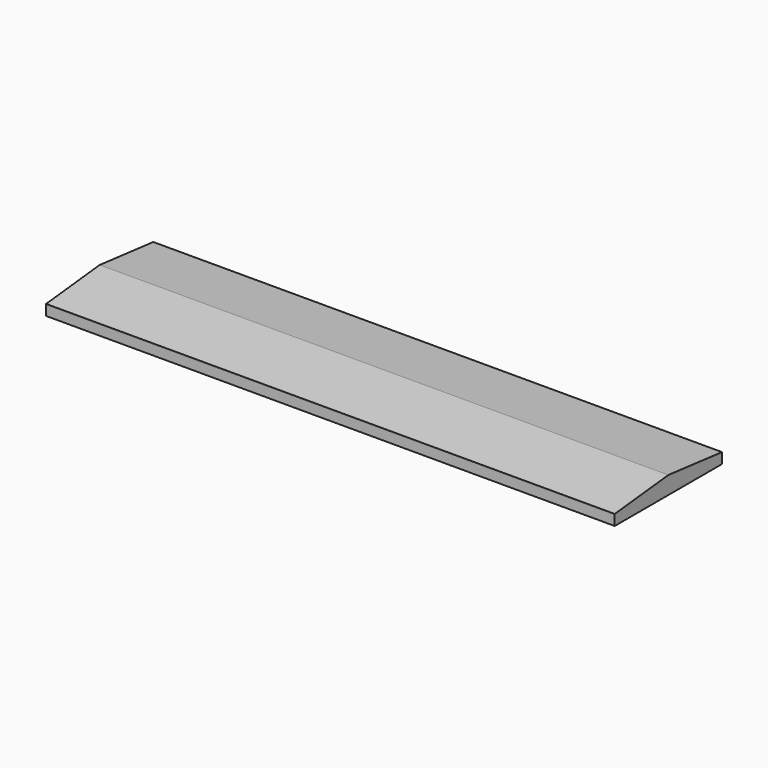
from build123d import *

# Parameters (mm, degrees)
F0_W          = 39250
F0_H          = 9250
F1_DEPTH      = 150
F2_W          = 39250
F2_H          = 9250
F2_W_2        = 38950
F2_H_2        = 8950
F3_DEPTH      = 570
F5_DEPTH      = 39250.001
F7_DEPTH      = 50
F7_DEPTH_BACK = 39300
F9_DEPTH      = 150
F11_DEPTH     = 150
F12_W         = 266.9223773158
F12_H         = 1000
F13_DEPTH     = 1220.2764139782
F14_W         = 44695.1484680176
F14_H         = 14306.3936233521
F14_W_2       = 39250
F14_H_2       = 9250
F15_DEPTH     = 1220.2764139782
F17_DEPTH     = 38950


with BuildPart() as f1:
    # F0 (on Top) → F1 (new body)
    with BuildSketch(Plane.XY):
        with Locations((19625, -4625)):
            Rectangle(F0_W, F0_H)
    extrude(amount=F1_DEPTH)

    # F2 (on face) → F3 (join)
    with BuildSketch(Plane.XY.offset(150)):
        with Locations((19625, -4625)):
            Rectangle(F2_W, F2_H)
        with Locations((19625, -4625)):
            Rectangle(F2_W_2, F2_H_2, mode=Mode.SUBTRACT)
    extrude(amount=F3_DEPTH)

    # F4 (on face) → F5 (cut, through all)
    with BuildSketch(Plane(origin=(0, 0, 0), x_dir=(0, -1, 0), z_dir=(-1, 0, 0))):
        Polygon((-659.6078069495, 614.5653377715), (4625, 1170), (1956.3378095627, 2374.1724491119), align=None)
        Polygon((7293.6621904373, 2374.1724491119), (4625, 1170), (9909.6078069495, 614.5653377715), align=None)
    extrude(amount=-F5_DEPTH, mode=Mode.SUBTRACT)

    # F8 (on face) → F9 (join)
    with BuildSketch(Plane.YZ.offset(39250)):
        Polygon((-8906.4640044002, 720), (-343.5359955999, 720), (-4625, 1170), align=None)
    extrude(amount=-F9_DEPTH)

    # F10 (on face) → F11 (join)
    with BuildSketch(Plane(origin=(0, 0, 0), x_dir=(0, -1, 0), z_dir=(-1, 0, 0))):
        Polygon((4625, 1170), (343.5359955998, 720), (8906.4640044001, 720), align=None)
    extrude(amount=-F11_DEPTH)


with BuildPart() as f7:
    # F6 (on face) → F7 (new body, two sides)
    with BuildSketch(Plane(origin=(0, 0, 0), x_dir=(0, -1, 0), z_dir=(-1, 0, 0))) as f7_sk:
        Polygon((-98.9790029993, 673.4897994786), (4625, 1170), (9348.9790029993, 673.4897994786), (9354.2054261627, 723.2158942471), (4625, 1220.2754139782), (-104.2054261627, 723.2158942471), align=None)
    extrude(amount=F7_DEPTH)
    extrude(f7_sk.sketch, amount=-F7_DEPTH_BACK)

    # F12 (on face) → F13 (cut, through all)
    with BuildSketch(Plane(origin=(0, 0, 0), x_dir=(1, 0, 0), z_dir=(0, 0, -1))):
        with Locations((-133.4611886579, 600)):
            Rectangle(F12_W, F12_H)
    extrude(amount=-F13_DEPTH, mode=Mode.SUBTRACT)

    # F14 (on face) → F15 (cut, through all)
    with BuildSketch(Plane(origin=(0, 0, 0), x_dir=(1, 0, 0), z_dir=(0, 0, -1))):
        with Locations((18414.8387908936, 3717.1730995178)):
            Rectangle(F14_W, F14_H)
        with Locations((19625, 4625)):
            Rectangle(F14_W_2, F14_H_2, mode=Mode.SUBTRACT)
    extrude(amount=-F15_DEPTH, mode=Mode.SUBTRACT)


with BuildPart() as f17:
    # F16 (on face) → F17 (new body, through all)
    with BuildSketch(Plane.YZ.offset(150)):
        Polygon((-9100, 150), (-150, 150), (-150, 699.6585471861), (-4625, 1170), (-9100, 699.6585471861), align=None)
    extrude(amount=F17_DEPTH)


solid = Compound([f1.part, f7.part, f17.part])
